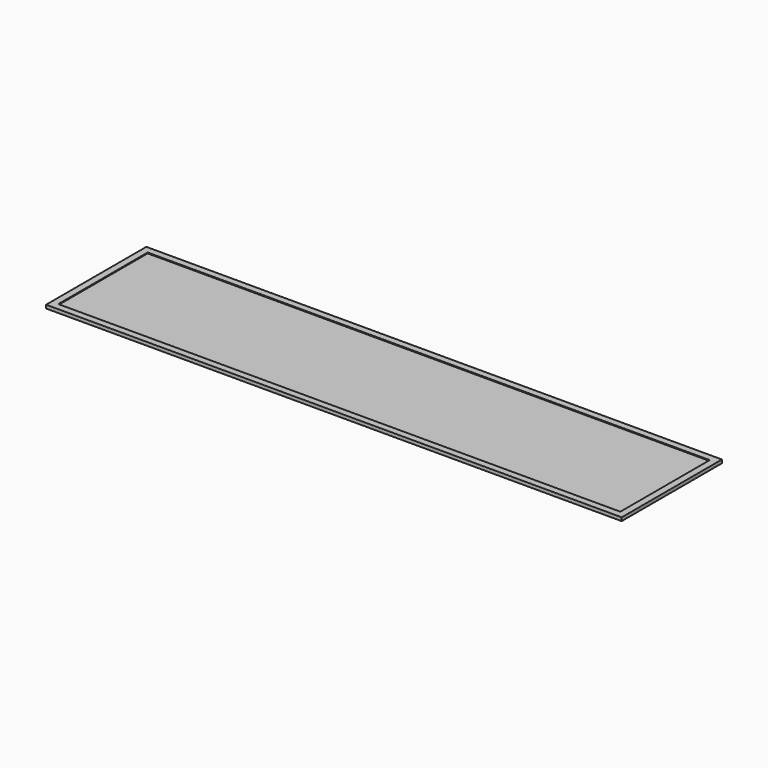
from build123d import *

# Parameters (mm, degrees)
F0_W     = 539.75
F0_H     = 117.475
F1_DEPTH = 3.175
F2_W     = 528.6375
F2_H     = 106.3625
F3_DEPTH = 1.5875
F5_DEPTH = 1.5875


with BuildPart() as f1:
    # F0 (on Top) → F1 (new body)
    with BuildSketch(Plane.XY):
        with Locations((269.875, 58.7375)):
            Rectangle(F0_W, F0_H)
        Polygon((6.35, 6.35), (6.35, 57.15), (6.35, 111.125), (533.4, 111.125), (533.4, 6.35), align=None, mode=Mode.SUBTRACT)
    extrude(amount=F1_DEPTH)



with BuildPart() as f3:
    # F2 (on Top) → F3 (new body)
    with BuildSketch(Plane.XY):
        with Locations((270.66875, 59.53125)):
            Rectangle(F2_W, F2_H)
    extrude(amount=F3_DEPTH)


with BuildPart() as f3_1:
    # F4: moved
    add(f3.part.moved(Location((-0.79375, -0.79375, 0.79375))))


with BuildPart() as f1_1:
    add(f1.part)
    # F5 (cut): a face of the model
    f5_faces = [f3_1.part.faces().sort_by_distance(p)[0] for p in [
        (269.875, 58.7375, 2.38125),
    ]]
    extrude(f5_faces, amount=-F5_DEPTH, mode=Mode.SUBTRACT)


solid = Compound([f3_1.part, f1_1.part])
